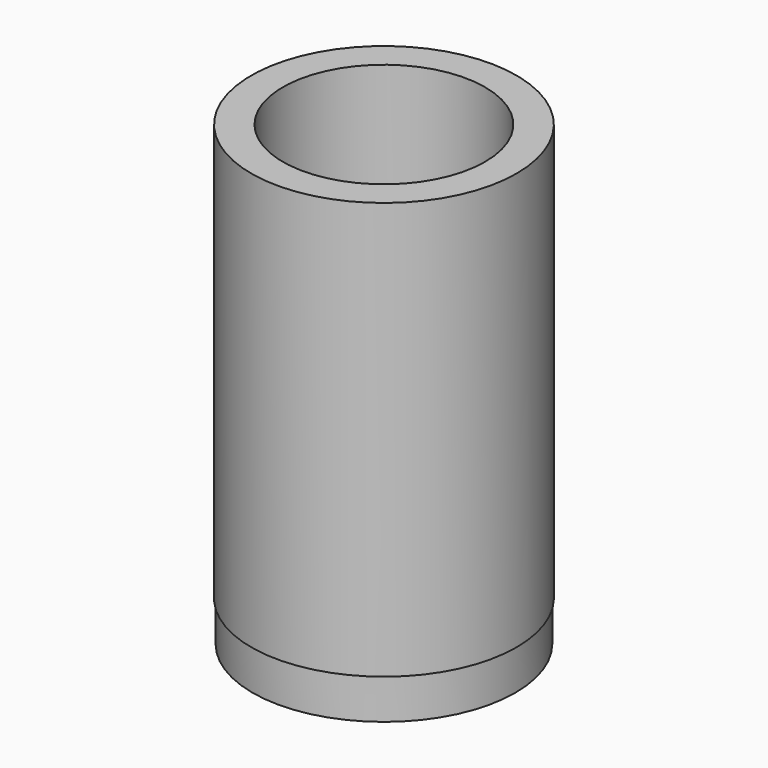
from build123d import *
from build123d import SkipClean  # not in build123d's __all__

# Parameters (mm, degrees)
F0_R     = 26
F1_DEPTH = 8
F2_R     = 26.25
F2_R_2   = 20
F3_DEPTH = 82.5


with BuildPart() as f1:
    # F0 (on Top) → F1 (new body)
    with BuildSketch(Plane.XY):
        Circle(F0_R)
        with BuildLine():
            ThreePointArc((7, 18.7349939952), (19.9390246123, -1.5605439791), (4, -19.5959179423))
            Line((4, -19.5959179423), (2.5, -16.9978417309))
            ThreePointArc((2.5, -16.9978417309), (0, -17.1816769299), (-2.5, -16.9978417309))
            Line((-2.5, -16.9978417309), (-4, -19.5959179423))
            ThreePointArc((-4, -19.5959179423), (-19.9390246123, -1.5605439791), (-7, 18.7349939952))
            Line((-7, 18.7349939952), (-5, 16.4989260177))
            ThreePointArc((-5, 16.4989260177), (0, 17.2452185999), (5, 16.4989260177))
            Line((5, 16.4989260177), (7, 18.7349939952))
        make_face(mode=Mode.SUBTRACT)
    extrude(amount=F1_DEPTH)

    # F2 (on face) → F3 (join)
    with BuildSketch(Plane.XY.offset(8)):
        Circle(F2_R)
        Circle(F2_R_2, mode=Mode.SUBTRACT)
    with SkipClean():  # cleaning this boolean's faces spoils the solid; the shape is the same uncleaned
        extrude(amount=F3_DEPTH)


solid = f1.part
